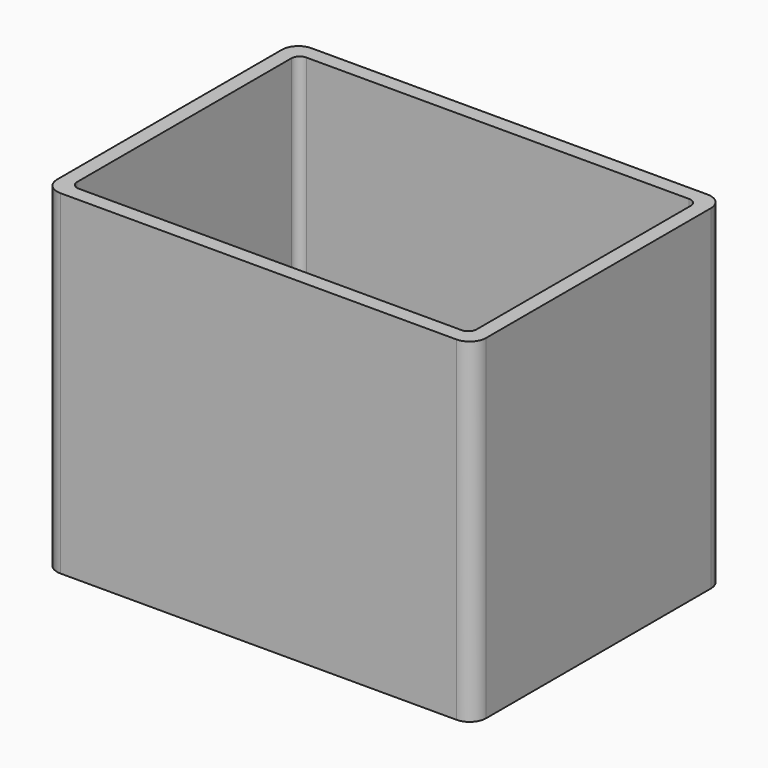
from build123d import *

# Parameters (mm, degrees)
F1_DEPTH = 40.64
F3_DEPTH = 38.608
F5_DEPTH = 4.7752
F6_R     = 1.35255
F7_DEPTH = 4.7752


# Not quite as in the source:
# - a feature names something its author has since deleted; it is built from what else it names


with BuildPart() as f1:
    # F0 (on Top) → F1 (new body)
    with BuildSketch(Plane.XY):
        with BuildLine():
            ThreePointArc((0, 2), (0.5857864376, 0.5857864376), (2, 0))
            Line((2, 0), (50.07, 0))
            ThreePointArc((50.07, 0), (51.4842135624, 0.5857864376), (52.07, 2))
            Line((52.07, 2), (52.07, 36.1))
            ThreePointArc((52.07, 36.1), (51.4842135624, 37.5142135624), (50.07, 38.1))
            Line((50.07, 38.1), (2, 38.1))
            ThreePointArc((2, 38.1), (0.5857864376, 37.5142135624), (0, 36.1))
            Line((0, 36.1), (0, 2))
        make_face()
    extrude(amount=F1_DEPTH)

    # F2 (on face) → F3 (cut)
    with BuildSketch(Plane.XY.offset(40.64)):
        with BuildLine():
            Line((49.27, 36.3), (2.8, 36.3))
            ThreePointArc((2.8, 36.3), (2.0928932188, 36.0071067812), (1.8, 35.3))
            Line((1.8, 35.3), (1.8, 2.8))
            ThreePointArc((1.8, 2.8), (2.0928932188, 2.0928932188), (2.8, 1.8))
            Line((2.8, 1.8), (49.27, 1.8))
            ThreePointArc((49.27, 1.8), (49.9771067812, 2.0928932188), (50.27, 2.8))
            Line((50.27, 2.8), (50.27, 35.3))
            ThreePointArc((50.27, 35.3), (49.9771067812, 36.0071067812), (49.27, 36.3))
        make_face()
    extrude(amount=-F3_DEPTH, mode=Mode.SUBTRACT)

    # F4 (on face) → F5 (join)
    with BuildSketch(Plane(origin=(0, 0, 0), x_dir=(1, 0, 0), z_dir=(0, 0, -1))):
        with BuildLine():
            ThreePointArc((52.07, -2), (51.4842135624, -0.5857864376), (50.07, 0))
            Line((50.07, 0), (46.26, 0))
            Line((46.26, 0), (46.26, -2))
            ThreePointArc((46.26, -2), (47.3759231637, -4.6940768363), (50.07, -5.81))
            Line((50.07, -5.81), (52.07, -5.81))
            Line((52.07, -5.81), (52.07, -2))
        make_face()
        with BuildLine():
            Line((46.26, -36.1), (46.26, -38.1))
            Line((46.26, -38.1), (50.07, -38.1))
            ThreePointArc((50.07, -38.1), (51.4842135624, -37.5142135624), (52.07, -36.1))
            Line((52.07, -36.1), (52.07, -32.29))
            Line((52.07, -32.29), (50.07, -32.29))
            ThreePointArc((50.07, -32.29), (47.3759231637, -33.4059231637), (46.26, -36.1))
        make_face()
        with BuildLine():
            ThreePointArc((5.81, -36.1), (4.6940768363, -33.4059231637), (2, -32.29))
            Line((2, -32.29), (0, -32.29))
            Line((0, -32.29), (0, -36.1))
            ThreePointArc((0, -36.1), (0.5857864376, -37.5142135624), (2, -38.1))
            Line((2, -38.1), (5.81, -38.1))
            Line((5.81, -38.1), (5.81, -36.1))
        make_face()
        with BuildLine():
            Line((5.81, 0), (2, 0))
            ThreePointArc((2, 0), (0.5857864376, -0.5857864376), (0, -2))
            Line((0, -2), (0, -5.81))
            Line((0, -5.81), (2, -5.81))
            ThreePointArc((2, -5.81), (4.6940768363, -4.6940768363), (5.81, -2))
            Line((5.81, -2), (5.81, 0))
        make_face()
    extrude(amount=-F5_DEPTH)

    # F6 (on face) → F7 (cut, through all)
    with BuildSketch(Plane(origin=(0, 0, 0), x_dir=(1, 0, 0), z_dir=(0, 0, -1))):
        with Locations((48.7198709242, -3.3501290758)):
            Circle(F6_R)
        with Locations((3.3501290758, -3.3501290758)):
            Circle(F6_R)
        with Locations((3.3501290758, -34.7498709242)):
            Circle(F6_R)
        with Locations((48.7198709242, -34.7498709242)):
            Circle(F6_R)
    extrude(amount=-F7_DEPTH, mode=Mode.SUBTRACT)


solid = f1.part
